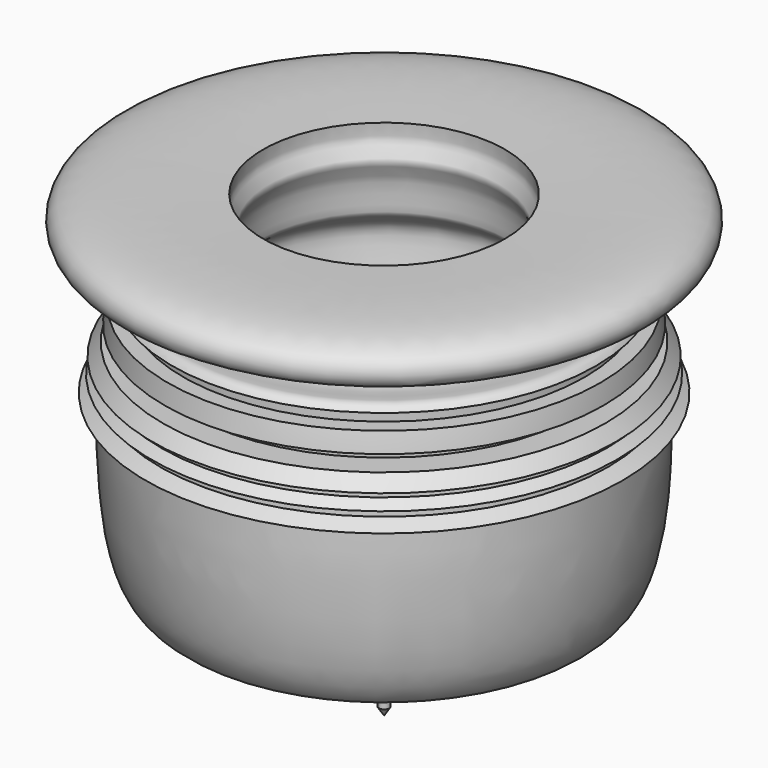
from build123d import *


# Not quite as in the source:
# - a feature names something its author has since deleted; it is built from what else it names


with BuildPart() as f1:
    # F0 (on Front) → F1 (revolve)
    with BuildSketch(Plane.XZ):
        with BuildLine():
            add(Edge.make_bspline(
                [(5.4458385124, 15.6634841114), (5.4426992502, 15.3170629144), (5.5833172951, 14.9657589831), (4.9596099598, 14.245520909), (5.589108727, 13.552596485), (5.5427438151, 12.2448683469), (5.6460651453, 11.7434094436), (7.0795890557, 11.0663661868), (6.8995157368, 9.5273460061), (6.1006779938, 5.4868925152), (6.051238002, 3.1345104864), (5.932182655, 2.7828202265), (6.2817245892, 2.1861518437), (5.4458385124, 2.221473027)],
                knots=[0, 0, 0, 0, 0.072396743, 0.1442037942, 0.2209263229, 0.3160691563, 0.3750536466, 0.4718485484, 0.5710183822, 0.748087412, 0.87486103, 0.9255425144, 1, 1, 1, 1], degree=3))
            Line((5.4458385124, 2.221473027), (1.8570761203, 2.221473027))
            Line((1.8570761203, 2.221473027), (0, 10))
            Line((0, 10), (0, 2.221473027))
            Line((0, 2.221473027), (0, 0))
            Line((0, 0), (0, -5.0041857176))
            Line((0, -5.0041857176), (0.2343666443, -4.636623742))
            Line((0.2343666443, -4.636623742), (0.2343666443, -3.249527188))
            Line((0.2343666443, -3.249527188), (0.621939157, -4.0287858868))
            Line((0.621939157, -4.0287858868), (0.7666355889, -3.8018555294))
            Line((0.7666355889, -3.8018555294), (0.621939157, -2.5020928588))
            Line((0.621939157, -2.5020928588), (1.2546253335, -3.0365312868))
            Line((1.2546253335, -3.0365312868), (3.190793097, 0))
            add(Edge.make_bspline(
                [(3.190793097, 0), (4.1430603402, 0), (5.4306340505, 0), (6.3829012937, 0)],
                knots=[0, 0, 0, 0, 3.1921081967, 3.1921081967, 3.1921081967, 3.1921081967], degree=3))
            add(Edge.make_bspline(
                [(6.3829012937, 0), (7.4278653987, -0.23657947), (9.8578113438, -0.7863606467), (10.1923974106, 5.0783004491), (10.0948148285, 7.8022954985)],
                knots=[0, 0, 0, 0, 0.1203087356, 0.2726129152, 0.2726129152, 0.2726129152, 0.2726129152], degree=3))
            add(Edge.make_bspline(
                [(10.0948148285, 7.8022954985), (10.0909108914, 7.9112729922), (10.0865515904, 8.0193662132), (10.0817605853, 8.126411587)],
                knots=[0.2726129152, 0.2726129152, 0.2726129152, 0.2726129152, 0.2787060716, 0.2787060716, 0.2787060716, 0.2787060716], degree=3))
            add(Edge.make_bspline(
                [(10.0817605853, 8.126411587), (10.0753819982, 8.2689282881), (10.0682381992, 8.4095876395), (10.0603850232, 8.5480036214)],
                knots=[0.2787060716, 0.2787060716, 0.2787060716, 0.2787060716, 0.2868183002, 0.2868183002, 0.2868183002, 0.2868183002], degree=3))
            add(Edge.make_bspline(
                [(10.0603850232, 8.5480036214), (10.0542134435, 8.6567806661), (10.047603758, 8.7641722227), (10.0405830661, 8.8699909372)],
                knots=[0.2868183002, 0.2868183002, 0.2868183002, 0.2868183002, 0.2931934618, 0.2931934618, 0.2931934618, 0.2931934618], degree=3))
            add(Edge.make_bspline(
                [(10.0405830661, 8.8699909372), (10.0323413803, 8.9942129683), (10.0235332977, 9.116267508), (10.0142026582, 9.2358514667)],
                knots=[0.2931934618, 0.2931934618, 0.2931934618, 0.2931934618, 0.3006773509, 0.3006773509, 0.3006773509, 0.3006773509], degree=3))
            add(Edge.make_bspline(
                [(10.0142026582, 9.2358514667), (9.998409287, 9.4382635131), (9.9811187828, 9.6335973083), (9.9625437439, 9.8203830421)],
                knots=[0.3006773509, 0.3006773509, 0.3006773509, 0.3006773509, 0.3133448468, 0.3133448468, 0.3133448468, 0.3133448468], degree=3))
            Line((9.9625437439, 9.8203830421), (8.8382373747, 9.8203830421))
            Line((8.8382373747, 9.8203830421), (8.8382373747, 10.5026598325))
            Line((8.8382373747, 10.5026598325), (9.8840050008, 10.5026598325))
            add(Edge.make_bspline(
                [(9.8840050008, 10.5026598325), (9.8399129011, 10.8341320589), (9.7916038683, 11.1218449708), (9.7408970609, 11.3532217219)],
                knots=[0.3298224991, 0.3298224991, 0.3298224991, 0.3298224991, 0.3557321119, 0.3557321119, 0.3557321119, 0.3557321119], degree=3))
            Line((9.7408970609, 11.3532217219), (9.0419609572, 11.3532217219))
            Line((9.0419609572, 11.3532217219), (9.0419609572, 11.9569053175))
            Line((9.0419609572, 11.9569053175), (9.5405176931, 11.9569053175))
            add(Edge.make_bspline(
                [(9.5405176931, 11.9569053175), (9.4293821341, 12.1519504238), (9.0230360003, 12.3606776001), (7.4758860135, 11.7807017496), (6.7849650417, 14.8787052356), (11.7933896772, 13.2037578467), (12.1667597112, 15.9992973155), (8.5096708179, 15.7319407269), (5.4458385124, 15.6634841114)],
                knots=[0.3863578023, 0.3863578023, 0.3863578023, 0.3863578023, 0.4304708956, 0.5144757413, 0.6031680217, 0.7446415244, 0.8204432659, 1, 1, 1, 1], degree=3))
        make_face()
        with BuildLine():
            Line((10.4301804677, 9.2358514667), (9.9625437439, 9.8203830421))
            add(Edge.make_bspline(
                [(10.0142026582, 9.2358514667), (9.998409287, 9.4382635131), (9.9811187828, 9.6335973083), (9.9625437439, 9.8203830421)],
                knots=[0.3006773509, 0.3006773509, 0.3006773509, 0.3006773509, 0.3133448468, 0.3133448468, 0.3133448468, 0.3133448468], degree=3))
            Line((10.0142026582, 9.2358514667), (10.4301804677, 9.2358514667))
        make_face()
        with BuildLine():
            Line((10.479958728, 8.5480036214), (10.0405830661, 8.8699909372))
            add(Edge.make_bspline(
                [(10.0603850232, 8.5480036214), (10.0542134435, 8.6567806661), (10.047603758, 8.7641722227), (10.0405830661, 8.8699909372)],
                knots=[0.2868183002, 0.2868183002, 0.2868183002, 0.2868183002, 0.2931934618, 0.2931934618, 0.2931934618, 0.2931934618], degree=3))
            Line((10.0603850232, 8.5480036214), (10.479958728, 8.5480036214))
        make_face()
        with BuildLine():
            Line((10.7356701046, 7.8022954985), (10.0817605853, 8.126411587))
            add(Edge.make_bspline(
                [(10.0948148285, 7.8022954985), (10.0909108914, 7.9112729922), (10.0865515904, 8.0193662132), (10.0817605853, 8.126411587)],
                knots=[0.2726129152, 0.2726129152, 0.2726129152, 0.2726129152, 0.2787060716, 0.2787060716, 0.2787060716, 0.2787060716], degree=3))
            Line((10.0948148285, 7.8022954985), (10.7356701046, 7.8022954985))
        make_face()
    revolve(axis=Axis((0, 0, 10), (0, 0, -1)))


solid = f1.part
